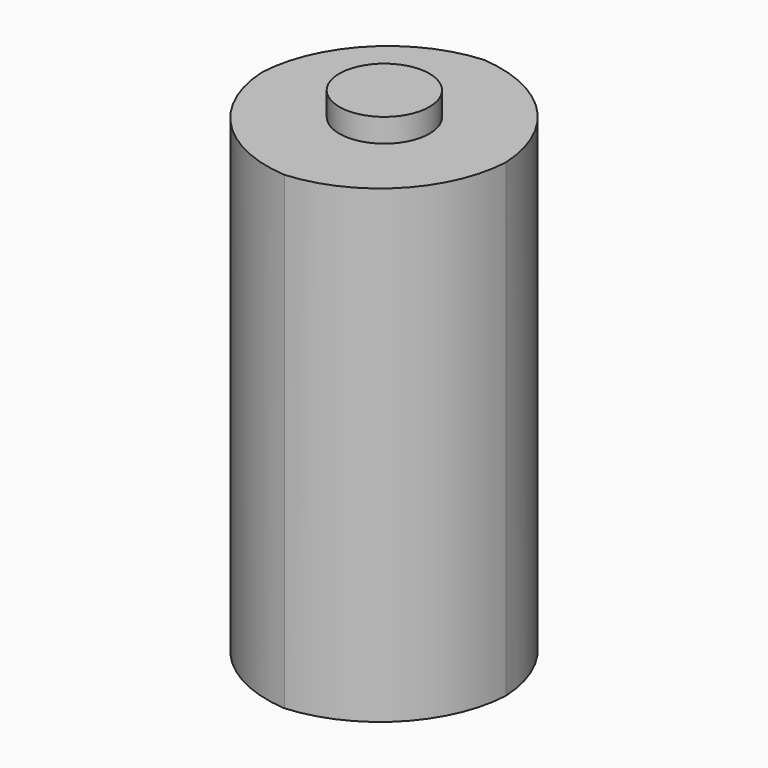
from build123d import *

# Parameters (mm, degrees)
F0_W        = 13
F0_H        = 25
F1_DEPTH    = 13.3
F2_T1_DEPTH = 60
F3_R        = 2.3988819555
F4_DEPTH    = 12.2


# Not quite as in the source:
# - a fillet or chamfer that OpenCascade refuses, or shapes differently, is made with other operations: its cross-section is extruded or revolved along the edge and cut away or added
# - a feature names something its author has since deleted; it is built from what else it names


with BuildPart() as f1:
    # F0 (on Front) → F1 (new body)
    with BuildSketch(Plane.XZ):
        with Locations((0, -1.5561378314)):
            Rectangle(F0_W, F0_H)
    extrude(amount=F1_DEPTH)

    # F2: fillet of radius 7 on 4 edges, made by hand

    # F2_s2 → F2_t1 (cut)
    with BuildSketch(Plane.XY.offset(-31.5561378314)):
        with BuildLine():
            ThreePointArc((6.5, -6.3), (4.4497474683, -11.2497474683), (-0.5, -13.3))
            Line((-0.5, -13.3), (6.5, -13.3))
            Line((6.5, -13.3), (6.5, -6.3))
        make_face()
        with BuildLine():
            ThreePointArc((6.5, -7), (4.4497474683, -2.0502525317), (-0.5, 0))
            Line((-0.5, 0), (6.5, 0))
            Line((6.5, 0), (6.5, -7))
        make_face()
        with BuildLine():
            ThreePointArc((-6.5, -7), (-4.4497474683, -2.0502525317), (0.5, 0))
            Line((0.5, 0), (-6.5, 0))
            Line((-6.5, 0), (-6.5, -7))
        make_face()
        with BuildLine():
            ThreePointArc((-6.5, -6.3), (-4.4497474683, -11.2497474683), (0.5, -13.3))
            Line((0.5, -13.3), (-6.5, -13.3))
            Line((-6.5, -13.3), (-6.5, -6.3))
        make_face()
    extrude(amount=F2_T1_DEPTH, mode=Mode.SUBTRACT)

    # F3 (on Top) → F4 (join)
    with BuildSketch(Plane.XY):
        with Locations((0, -6.6247042269)):
            Circle(F3_R)
    extrude(amount=F4_DEPTH)


solid = f1.part
